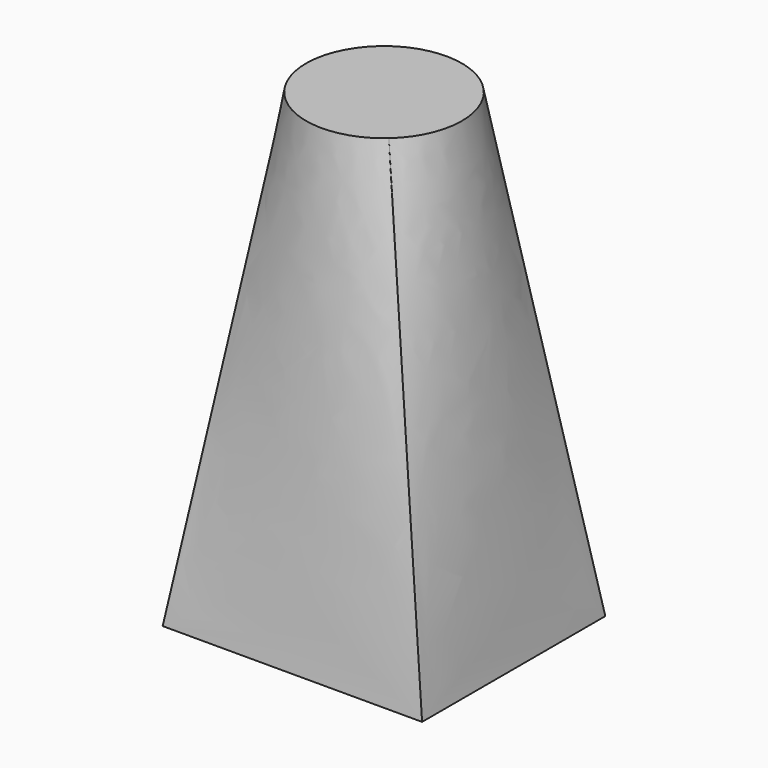
from build123d import *

# Parameters (mm, degrees)
F0_W = 70.7477629185
F0_H = 62.4708645046
F4_T = 2.54


# Not quite as in the source:
# - the arcs of a loft's sections are written as splines that run evenly, so that the points pair up as in the source's solid
# - a shell that OpenCascade refuses in one call is made with other operations: the cavity is built on its own and cut out


with BuildPart() as f3:
    # F0 (on Top) → F3 section 0
    with BuildSketch(Plane.XY):
        Rectangle(F0_W, F0_H)
    # F2 (on offset) → F3 section 1
    with BuildSketch(Plane.XY.offset(127)):
        with BuildLine():
            add(Edge.make_bspline(
                [(15.9351280148, 14.0708508936), (15.0141929774, 15.1138025832), (13.9905614763, 16.0660265425), (11.7771428565, 17.7525188473), (10.5874104689, 18.4867454911), (8.0875037404, 19.7090157679), (6.7773912146, 20.1970291779), (4.087066391, 20.9081062654), (2.7069206167, 21.13115236), (-0.0704346278, 21.3037099645), (-1.4675754224, 21.2532172075), (-4.2252288833, 20.8806240369), (-5.5856733611, 20.5585328366), (-8.2176499623, 19.6551074376), (-9.4891170049, 19.0737955781), (-11.8942713618, 17.6742560822), (-13.0278992039, 16.8560630523), (-14.0708508936, 15.9351280148)],
                knots=[0, 0, 0, 0, 0.125, 0.125, 0.25, 0.25, 0.375, 0.375, 0.5, 0.5, 0.625, 0.625, 0.75, 0.75, 0.875, 0.875, 1, 1, 1, 1], degree=3))
            add(Edge.make_bspline(
                [(-14.0708508936, 15.9351280148), (-15.1138025832, 15.0141929774), (-16.0660265425, 13.9905614763), (-17.7525188473, 11.7771428565), (-18.4867454911, 10.5874104689), (-19.7090157679, 8.0875037404), (-20.1970291779, 6.7773912146), (-20.9081062654, 4.087066391), (-21.13115236, 2.7069206167), (-21.3037099645, -0.0704346278), (-21.2532172075, -1.4675754224), (-20.8806240369, -4.2252288833), (-20.5585328366, -5.5856733611), (-19.6551074376, -8.2176499623), (-19.0737955781, -9.4891170049), (-17.6742560822, -11.8942713618), (-16.8560630523, -13.0278992039), (-15.9351280148, -14.0708508936)],
                knots=[0, 0, 0, 0, 0.125, 0.125, 0.25, 0.25, 0.375, 0.375, 0.5, 0.5, 0.625, 0.625, 0.75, 0.75, 0.875, 0.875, 1, 1, 1, 1], degree=3))
            add(Edge.make_bspline(
                [(-15.9351280148, -14.0708508936), (-15.0141929774, -15.1138025832), (-13.9905614763, -16.0660265425), (-11.7771428565, -17.7525188473), (-10.5874104689, -18.4867454911), (-8.0875037404, -19.7090157679), (-6.7773912146, -20.1970291779), (-4.087066391, -20.9081062654), (-2.7069206167, -21.13115236), (0.0704346278, -21.3037099645), (1.4675754224, -21.2532172075), (4.2252288833, -20.8806240369), (5.5856733611, -20.5585328366), (8.2176499623, -19.6551074376), (9.4891170049, -19.0737955781), (11.8942713618, -17.6742560822), (13.0278992039, -16.8560630523), (14.0708508936, -15.9351280148)],
                knots=[0, 0, 0, 0, 0.125, 0.125, 0.25, 0.25, 0.375, 0.375, 0.5, 0.5, 0.625, 0.625, 0.75, 0.75, 0.875, 0.875, 1, 1, 1, 1], degree=3))
            add(Edge.make_bspline(
                [(14.0708508936, -15.9351280148), (15.1138025832, -15.0141929774), (16.0660265425, -13.9905614763), (17.7525188473, -11.7771428565), (18.4867454911, -10.5874104689), (19.7090157679, -8.0875037404), (20.1970291779, -6.7773912146), (20.9081062654, -4.087066391), (21.13115236, -2.7069206167), (21.3037099645, 0.0704346278), (21.2532172075, 1.4675754224), (20.8806240369, 4.2252288833), (20.5585328366, 5.5856733611), (19.6551074376, 8.2176499623), (19.0737955781, 9.4891170049), (17.6742560822, 11.8942713618), (16.8560630523, 13.0278992039), (15.9351280148, 14.0708508936)],
                knots=[0, 0, 0, 0, 0.125, 0.125, 0.25, 0.25, 0.375, 0.375, 0.5, 0.5, 0.625, 0.625, 0.75, 0.75, 0.875, 0.875, 1, 1, 1, 1], degree=3))
        make_face()
    loft(ruled=True)

    # F4: shell of thickness 2.54, made by hand


with BuildPart() as f4_core1:
    # F4_t2: copy of F3
    add(f3.part)

    # the walls: a layer under each face that stays
    f4_faces = [f4_core1.faces().sort_by_distance(p)[0] for p in [
        (28.2956563107, -0.6591214972, 63.5),
        (0.6591214972, 26.2264317073, 63.5),
        (-28.2956563107, 0.6591214972, 63.5),
        (-0.6591214972, -26.2264317073, 63.5),
        (0, 0, 127),
    ]]
    thicken(f4_faces, amount=-F4_T, mode=Mode.SUBTRACT)


with BuildPart() as f3_1:
    add(f3.part)

    # what is left inside the walls is the cavity
    f4_cavity = [f4_core1.part.solids().sort_by_distance(p)[0] for p in [
        (-0.40374, -25.381852, 41.586065),
    ]]
    add(f4_cavity, mode=Mode.SUBTRACT)


solid = f3_1.part
